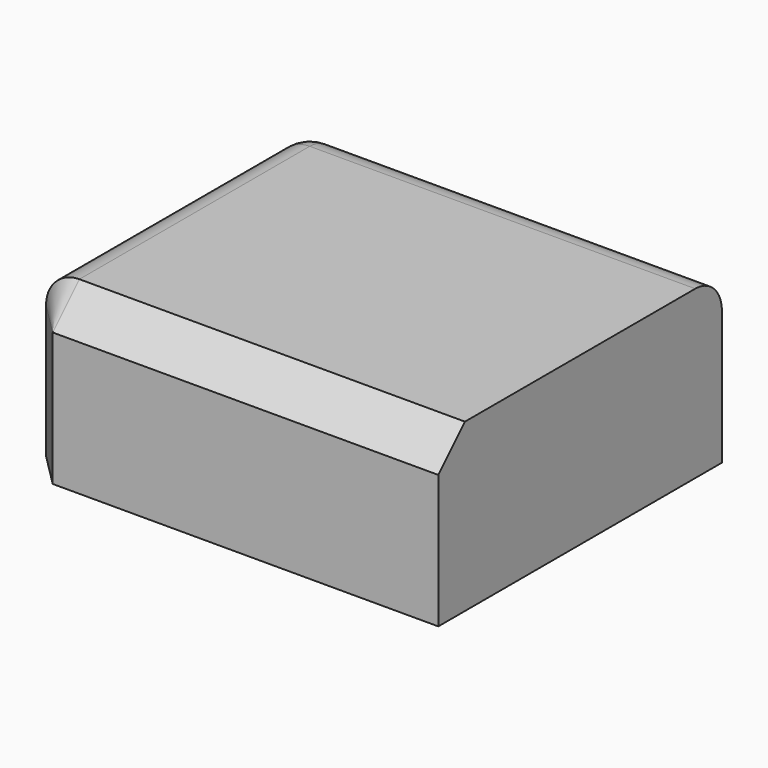
from build123d import *

# Parameters (mm, degrees)
F0_W     = 63.8230051845
F0_H     = 54.0183149278
F1_DEPTH = 25.4
F2_R     = 5.08
F3_R     = 5.08
F4_SIZE  = 5.07999


# Not quite as in the source:
# - a fillet or chamfer is up to 0.001 mm smaller than in the source, because OpenCascade refuses the exact size


with BuildPart() as f1:
    # F0 (on Top) → F1 (new body)
    with BuildSketch(Plane.XY):
        with Locations((-1.6649486497, -0.9249709547)):
            Rectangle(F0_W, F0_H)
    extrude(amount=-F1_DEPTH)

    # F2
    f2_edges = [f1.edges().sort_by_distance(p)[0] for p in [
        (-1.664949, 26.084187, 0),
    ]]
    fillet(f2_edges, radius=F2_R)

    # F3
    f3_edges = [f1.edges().sort_by_distance(p)[0] for p in [
        (-33.576451, -3.464971, 0),
    ]]
    fillet(f3_edges, radius=F3_R)

    # F4 (size 5.08 in the source; OpenCascade refuses exactly that, so slightly less here)
    f4_edges = [f1.edges().sort_by_distance(p)[0] for p in [
        (0.875051, -27.934128, 0),
    ]]
    chamfer(f4_edges, length=F4_SIZE)


solid = f1.part
